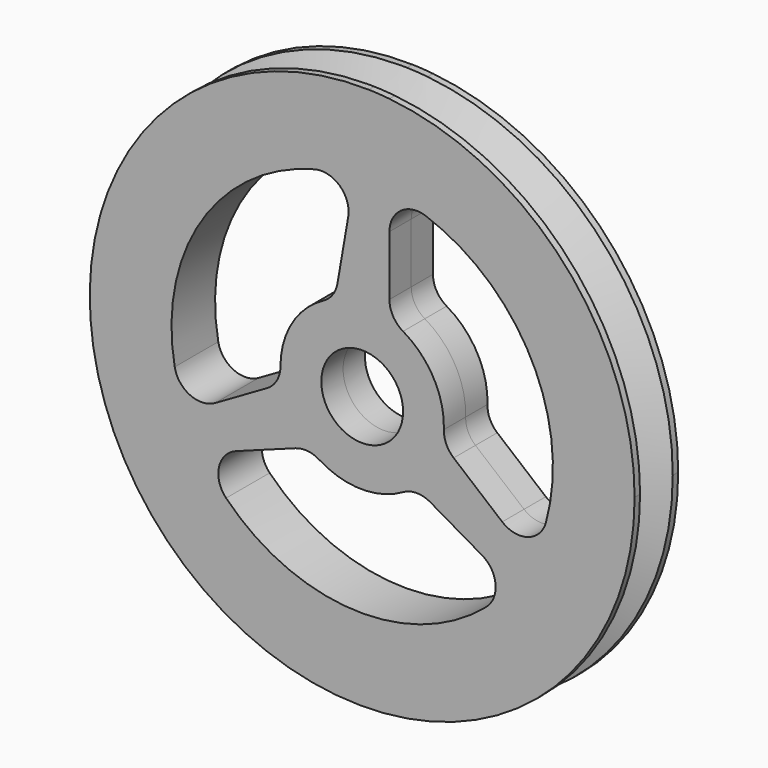
from build123d import *

# Parameters (mm, degrees)
F0_R     = 1.5
F1_DEPTH = 1


# Not quite as in the source:
# - ends of sketch curves that miss each other by under 0.0002 mm in the source are joined


with BuildPart() as f1:
    # F0 (on Front) → F1 (new body, symmetric)
    with BuildSketch(Plane.XZ):
        with BuildLine():
            ThreePointArc((0.2401150839, 9.9971168217), (-7.1554577365, -6.985658493), (10, 0))
            ThreePointArc((10, 0), (7.4161984871, 6.7082039325), (1, 9.9498743711))
            ThreePointArc((1, 9.9498743711), (0.6205086012, 9.9807298869), (0.2401150839, 9.9971168217))
        make_face()
        with BuildLine():
            ThreePointArc((4.5488093998, -5.3205575877), (-0.3054811817, -6.9933311982), (-4.9954209636, -4.90364858))
            ThreePointArc((-4.9954209636, -4.90364858), (-5.2574280938, -3.9837438223), (-4.6268502112, -3.2645470249))
            Line((-4.6268502112, -3.2645470249), (-2.4485091499, -2.4636990679))
            ThreePointArc((-2.4485091499, -2.4636990679), (-2.0029061262, -2.4073466036), (-1.5775862521, -2.551709548))
            ThreePointArc((-1.5775862521, -2.551709548), (-0.0451926266, -2.9996595851), (1.5, -2.5980762114))
            ThreePointArc((1.5, -2.5980762114), (2, -2.4641016151), (2.5, -2.5980762114))
            Line((2.5, -2.5980762114), (4.3989794856, -3.6944525285))
            ThreePointArc((4.3989794856, -3.6944525285), (4.8947614013, -4.4687262228), (4.5488093998, -5.3205575877))
        make_face(mode=Mode.SUBTRACT)
        with BuildLine():
            ThreePointArc((-0.9093714051, 3.3523206591), (-1.0833702513, 2.9382408884), (-1.4210521656, 2.6420845449))
            ThreePointArc((-1.4210521656, 2.6420845449), (-2.5751850901, 1.5389677552), (-3, 0))
            ThreePointArc((-3, 0), (-3.1339745962, -0.5), (-3.5, -0.8660254038))
            Line((-3.5, -0.8660254038), (-5.3989794856, -1.962401721))
            ThreePointArc((-5.3989794856, -1.962401721), (-6.3174111322, -2.0046246076), (-6.8821427332, -1.2791057034))
            ThreePointArc((-6.8821427332, -1.2791057034), (-5.9036618838, 3.7612200629), (-1.7489737597, 6.7779857471))
            ThreePointArc((-1.7489737597, 6.7779857471), (-0.8213093054, 6.5449381989), (-0.5137555498, 5.6392433348))
            Line((-0.5137555498, 5.6392433348), (-0.9093714051, 3.3523206591))
        make_face(mode=Mode.SUBTRACT)
        Circle(F0_R, mode=Mode.SUBTRACT)
        with BuildLine():
            Line((1, 3.4641016151), (1, 5.6568542495))
            ThreePointArc((1, 5.6568542495), (1.4226497308, 6.4733508304), (2.3333333333, 6.5996632911))
            ThreePointArc((2.3333333333, 6.5996632911), (6.2091430656, 3.2321111353), (6.7443947233, -1.8743371671))
            ThreePointArc((6.7443947233, -1.8743371671), (6.0787373992, -2.5611943766), (5.140605761, -2.3746963099))
            Line((5.140605761, -2.3746963099), (3.357880555, -0.8886215913))
            ThreePointArc((3.357880555, -0.8886215913), (3.0862763775, -0.5308942848), (2.9986384177, -0.090374997))
            ThreePointArc((2.9986384177, -0.090374997), (2.6203777167, 1.4606918299), (1.5, 2.5980762114))
            ThreePointArc((1.5, 2.5980762114), (1.1339745962, 2.9641016151), (1, 3.4641016151))
        make_face(mode=Mode.SUBTRACT)
    extrude(amount=F1_DEPTH, both=True)

    # F2 (on Right) → F3 (revolve, cut)
    with BuildSketch(Plane.YZ):
        Polygon((-0.75, 10), (0, 8.5), (0, 10), align=None)
        Polygon((0, 10), (0, 8.5), (0.75, 10), align=None)
    revolve(axis=Axis((0, 4.7748805955, 0), (0, 1, 0)), mode=Mode.SUBTRACT)


solid = f1.part
